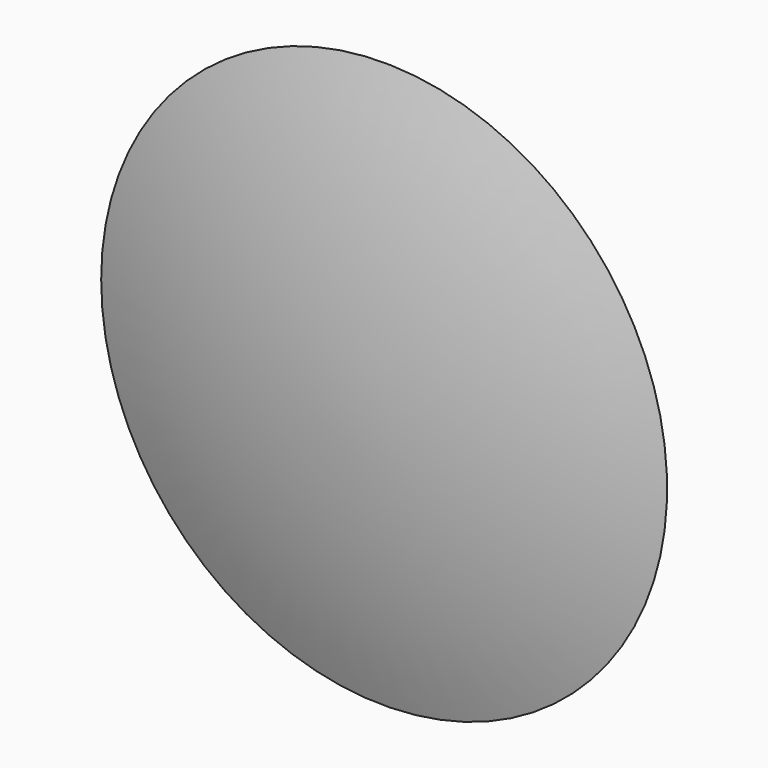
from build123d import *


# Not quite as in the source:
# - the program builds the solid bodies; features that only make, move or delete a surface that nothing else refers to are left out


with BuildPart() as f2:
    # F0 (on Top) → F2 (revolve)
    with BuildSketch(Plane.XY):
        with BuildLine():
            Line((0, -11.3592253257), (-8.2529602843, -11.3592253257))
            ThreePointArc((-8.2529602843, -11.3592253257), (-4.1779172362, -12.3375566039), (0, -12.6663658214))
            Line((0, -12.6663658214), (0, -11.3592253257))
        make_face()
    revolve(axis=Axis((0, -12.0127955735, 0), (0, 1, 0)))


solid = f2.part
